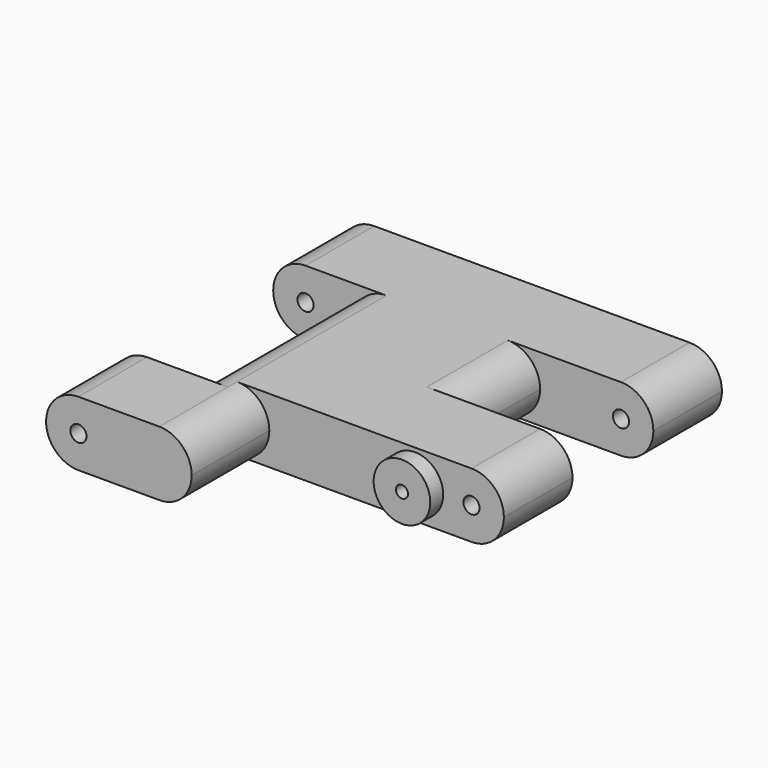
from build123d import *

# Parameters (mm, degrees)
F1_DEPTH = 8
F2_R     = 3.99999
F3_R     = 1
F4_DEPTH = 60
F6_R     = 3.99999
F5_R     = 3.5
F7_DEPTH = 2
F8_R     = 0.75
F9_DEPTH = 12


# Not quite as in the source:
# - a fillet or chamfer is up to 0.001 mm smaller than in the source, because OpenCascade refuses the exact size


with BuildPart() as f1:
    # F0 (on Top) → F1 (new body)
    with BuildSketch(Plane.XY):
        Polygon((-19.9077894302, -1.920078908), (-19.9077894302, -12.520078908), (-1.9077894302, -12.520078908), (-1.9077894302, -0.520078908), (27.0922105698, -0.520078908), (27.0922105698, 10.079921092), (13.0922105698, 10.079921092), (13.0922105698, 22.579921092), (27.0922105698, 22.579921092), (27.0922105698, 33.179921092), (-19.9077894302, 33.179921092), (-19.9077894302, 22.579921092), (-9.9077894302, 22.579921092), (-9.9077894302, -1.920078908), align=None)
    extrude(amount=F1_DEPTH)

    # F2 (radius 4 in the source; OpenCascade refuses exactly that, so slightly less here)
    f2_edges = [f1.edges().sort_by_distance(p)[0] for p in [
        (-19.907789, -7.220079, 8),
        (-19.907789, -7.220079, 0),
        (-1.907789, -6.520079, 8),
        (-1.907789, -6.520079, 0),
        (27.092211, 4.779921, 8),
        (27.092211, 4.779921, 0),
        (27.092211, 27.879921, 8),
        (27.092211, 27.879921, 0),
        (-19.907789, 27.879921, 8),
        (-19.907789, 27.879921, 0),
    ]]
    fillet(f2_edges, radius=F2_R)

    # F3 (on face) → F4 (cut)
    with BuildSketch(Plane(origin=(0, 33.179921092, 0), x_dir=(-1, 0, 0), z_dir=(0, 1, 0))):
        with Locations((-23.0922105698, 4)):
            Circle(F3_R)
        with Locations((15.9077894302, 4)):
            Circle(F3_R)
    extrude(amount=-F4_DEPTH, mode=Mode.SUBTRACT)

    # F6 (radius 4 in the source; OpenCascade refuses exactly that, so slightly less here)
    f6_edges = [f1.edges().sort_by_distance(p)[0] for p in [
        (-9.907789, 10.329921, 8),
        (-9.907789, 10.329921, 0),
        (13.092211, 16.329921, 8),
        (13.092211, 16.329921, 0),
    ]]
    fillet(f6_edges, radius=F6_R)

    # F5 (on face) → F7 (join)
    with BuildSketch(Plane.XZ.offset(0.520078908)):
        with Locations((16.0922105698, 4)):
            Circle(F5_R)
    extrude(amount=F7_DEPTH)

    # F8 (on face) → F9 (cut)
    with BuildSketch(Plane.XZ.offset(2.520078908)):
        with Locations((16.0922105698, 4)):
            Circle(F8_R)
    extrude(amount=-F9_DEPTH, mode=Mode.SUBTRACT)


solid = f1.part
